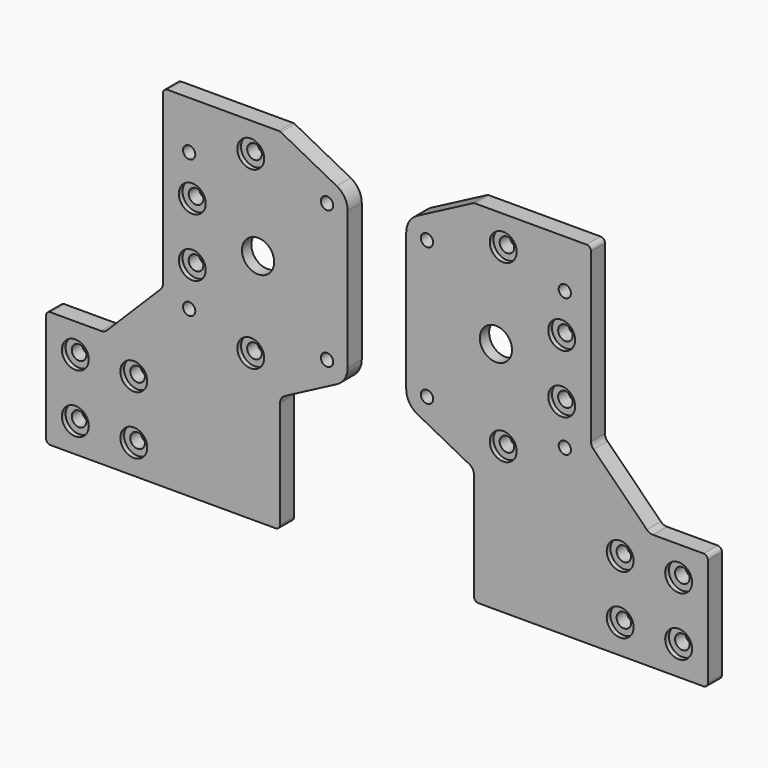
from build123d import *

# Parameters (mm, degrees)
F0_R     = 4.6
F0_R_2   = 2.1
F0_R_3   = 8.05
F0_R_4   = 2.5
F0_R_5   = 5.5
F1_DEPTH = 6
F2_DEPTH = 1.6
F3_START = -4
F3_DEPTH = 2
F4_R     = 1.5
F5_R     = 3


# Not quite as in the source:
# - a feature names something its author has since deleted; it is built from what else it names


with BuildPart() as f1:
    # F0 (on Front) → F1 (new body)
    with BuildSketch(Plane.XZ):
        with BuildLine():
            Line((13.17, -23.57), (13.17, 23.57))
            ThreePointArc((13.17, 23.57), (12.144361275, 27.2458856213), (9.3637647604, 29.859762611))
            Line((9.3637647604, 29.859762611), (-10, 40))
            Line((-10, 40), (-50, 40))
            Line((-50, 40), (-50, -20))
            Line((-50, -20), (-70, -40))
            Line((-70, -40), (-90, -40))
            Line((-90, -40), (-90, -80))
            Line((-90, -80), (-10, -80))
            Line((-10, -80), (-10, -40))
            Line((-10, -40), (9.3637647604, -29.859762611))
            ThreePointArc((9.3637647604, -29.859762611), (12.144361275, -27.2458856213), (13.17, -23.57))
        make_face()
        with Locations((-80, -70)):
            Circle(F0_R, mode=Mode.SUBTRACT)
        with Locations((-60, -70)):
            Circle(F0_R, mode=Mode.SUBTRACT)
        with Locations((-80, -50)):
            Circle(F0_R, mode=Mode.SUBTRACT)
        with Locations((-60, -50)):
            Circle(F0_R, mode=Mode.SUBTRACT)
        with Locations((-41.07, -23.57)):
            Circle(F0_R_2, mode=Mode.SUBTRACT)
        with Locations((-20, -30)):
            Circle(F0_R, mode=Mode.SUBTRACT)
        with Locations((6.07, -23.57)):
            Circle(F0_R_2, mode=Mode.SUBTRACT)
        with Locations((-40, -10)):
            Circle(F0_R, mode=Mode.SUBTRACT)
        with Locations((-40, 10)):
            Circle(F0_R, mode=Mode.SUBTRACT)
        with Locations((-41.07, 23.57)):
            Circle(F0_R_2, mode=Mode.SUBTRACT)
        with Locations((-17.5, 0)):
            Circle(F0_R_3, mode=Mode.SUBTRACT)
        with Locations((-20, 30)):
            Circle(F0_R, mode=Mode.SUBTRACT)
        with Locations((6.07, 23.57)):
            Circle(F0_R_2, mode=Mode.SUBTRACT)
        with Locations((-80, -50)):
            Circle(F0_R)
        with Locations((-80, -50)):
            Circle(F0_R_4, mode=Mode.SUBTRACT)
        with Locations((-80, -70)):
            Circle(F0_R)
        with Locations((-80, -70)):
            Circle(F0_R_4, mode=Mode.SUBTRACT)
        with Locations((-60, -50)):
            Circle(F0_R)
        with Locations((-60, -50)):
            Circle(F0_R_4, mode=Mode.SUBTRACT)
        with Locations((-60, -70)):
            Circle(F0_R)
        with Locations((-60, -70)):
            Circle(F0_R_4, mode=Mode.SUBTRACT)
        with Locations((-20, -30)):
            Circle(F0_R)
        with Locations((-20, -30)):
            Circle(F0_R_4, mode=Mode.SUBTRACT)
        with Locations((-40, -10)):
            Circle(F0_R)
        with Locations((-40, -10)):
            Circle(F0_R_4, mode=Mode.SUBTRACT)
        with Locations((-17.5, 0)):
            Circle(F0_R_3)
        with Locations((-17.5, 0)):
            Circle(F0_R_5, mode=Mode.SUBTRACT)
        with Locations((-40, 10)):
            Circle(F0_R)
        with Locations((-40, 10)):
            Circle(F0_R_4, mode=Mode.SUBTRACT)
        with Locations((-20, 30)):
            Circle(F0_R)
        with Locations((-20, 30)):
            Circle(F0_R_4, mode=Mode.SUBTRACT)
    extrude(amount=-F1_DEPTH)

    # F0 (on Front) → F2 (cut)
    with BuildSketch(Plane.XZ):
        with Locations((-80, -70)):
            Circle(F0_R)
        with Locations((-80, -70)):
            Circle(F0_R_4, mode=Mode.SUBTRACT)
        with Locations((-80, -50)):
            Circle(F0_R)
        with Locations((-80, -50)):
            Circle(F0_R_4, mode=Mode.SUBTRACT)
        with Locations((-60, -50)):
            Circle(F0_R)
        with Locations((-60, -50)):
            Circle(F0_R_4, mode=Mode.SUBTRACT)
        with Locations((-60, -70)):
            Circle(F0_R)
        with Locations((-60, -70)):
            Circle(F0_R_4, mode=Mode.SUBTRACT)
        with Locations((-20, -30)):
            Circle(F0_R)
        with Locations((-20, -30)):
            Circle(F0_R_4, mode=Mode.SUBTRACT)
        with Locations((-40, -10)):
            Circle(F0_R)
        with Locations((-40, -10)):
            Circle(F0_R_4, mode=Mode.SUBTRACT)
        with Locations((-40, 10)):
            Circle(F0_R)
        with Locations((-40, 10)):
            Circle(F0_R_4, mode=Mode.SUBTRACT)
        with Locations((-20, 30)):
            Circle(F0_R)
        with Locations((-20, 30)):
            Circle(F0_R_4, mode=Mode.SUBTRACT)
    extrude(amount=-F2_DEPTH, mode=Mode.SUBTRACT)

    # F0 (on Front) → F3 (cut)
    with BuildSketch(Plane.XZ.offset(F3_START)):
        with Locations((-17.5, 0)):
            Circle(F0_R_3)
        with Locations((-17.5, 0)):
            Circle(F0_R_5, mode=Mode.SUBTRACT)
    extrude(amount=-F3_DEPTH, mode=Mode.SUBTRACT)

    # F4
    f4_edges = [f1.edges().sort_by_distance(p)[0] for p in [
        (-50, 3, 40),
        (-10, 3, 40),
        (-90, 3, -40),
        (-10, 3, -80),
        (-90, 3, -80),
    ]]
    fillet(f4_edges, radius=F4_R)

    # F5
    f5_edges = [f1.edges().sort_by_distance(p)[0] for p in [
        (-50, 3, -20),
        (-70, 3, -40),
        (-10, 3, -40),
    ]]
    fillet(f5_edges, radius=F5_R)


with BuildPart() as f6_1:
    # F6: instance of F1
    add(f1.part.mirror(Plane(origin=(13.17, 3, 0), x_dir=(0, 1, 0), z_dir=(1, 0, 0))))


with BuildPart() as f6_1_1:
    # F7: moved
    add(f6_1.part.moved(Location((20, 0, 0))))


solid = Compound([f1.part, f6_1_1.part])
